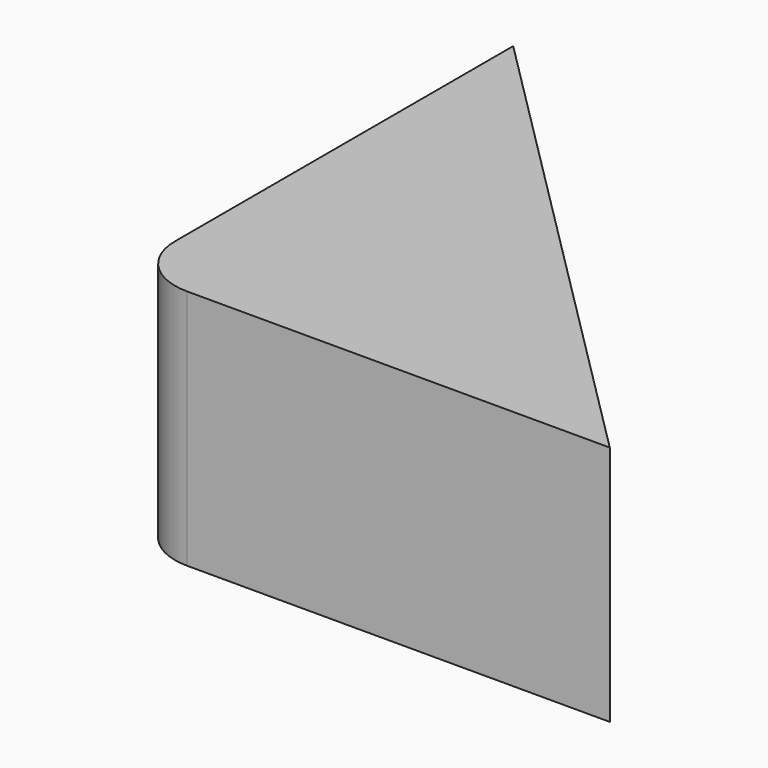
from build123d import *

# Parameters (mm, degrees)
F0_W        = 40
F0_H        = 40
F1_DEPTH    = 20
F2_T        = -2
F3_T1_DEPTH = 207.7346390373
F4_R        = 5


# Not quite as in the source:
# - a fillet or chamfer that OpenCascade refuses, or shapes differently, is made with other operations: its cross-section is extruded or revolved along the edge and cut away or added


with BuildPart() as f1:
    # F0 (on Top) → F1 (new body)
    with BuildSketch(Plane.XY):
        Rectangle(F0_W, F0_H)
    extrude(amount=F1_DEPTH)

    # F2
    f2_openings = [f1.faces().sort_by_distance(p)[0] for p in [
        (20, 0, 10),
        (0, 20, 10),
    ]]
    offset(amount=F2_T, openings=f2_openings)

    # F3: chamfer of 40 on 6 edges, made by hand

    # F3_s2 → F3_t1 (cut)
    with BuildSketch(Plane.XY.offset(-102.8673195186)):
        Polygon((20, -20), (-20, 20), (20, 20), align=None)
    extrude(amount=F3_T1_DEPTH, mode=Mode.SUBTRACT)

    # F4
    f4_edges = [f1.edges().sort_by_distance(p)[0] for p in [
        (-20, -20, 10),
    ]]
    fillet(f4_edges, radius=F4_R)


solid = f1.part
